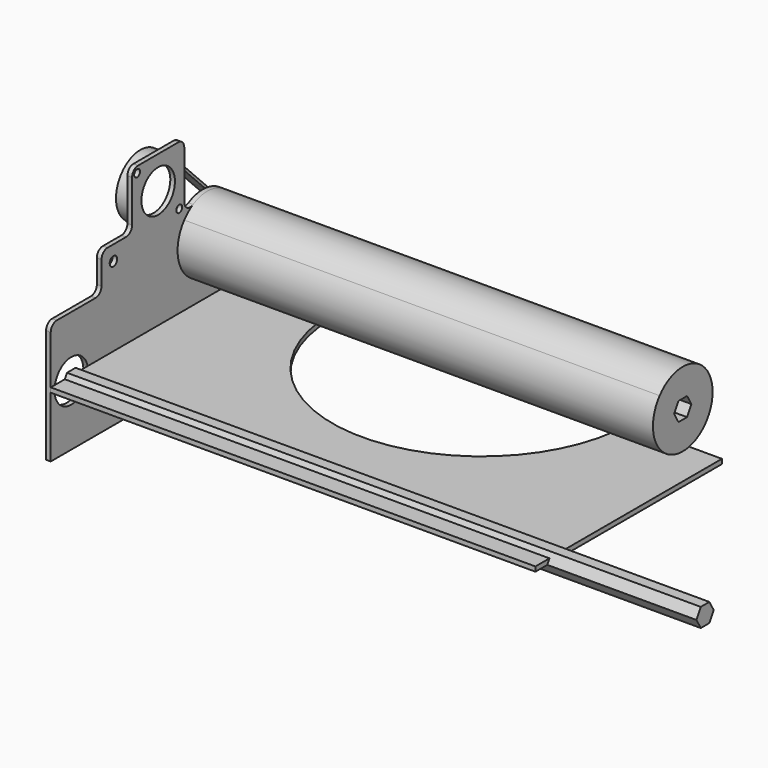
from build123d import *

# Parameters (mm, degrees)
F0_W     = 17.6947293282
F0_H     = 38.2016
F0_W_2   = 6.35
F0_H_2   = 28.575
F1_DEPTH = 3.175
F2_R     = 3.175
F2_R_2   = 2.4892
F2_R_3   = 14.2875
F3_DEPTH = 3.175
F4_R     = 14.2875
F5_DEPTH = 323.85
F6_DEPTH = 431.8
F8_DEPTH = 9
F9_R     = 5.08


# Not quite as in the source:
# - a feature names something its author has since deleted; it is built from what else it names


with BuildPart() as f1:
    # F0 (on Top) → F1 (new body)
    with BuildSketch(Plane.XY):
        with BuildLine():
            ThreePointArc((-90.5710140925, 31.75), (-98.622453308, 53.3708723969), (-101.5883780415, 76.2508))
            Line((-101.5883780415, 76.2508), (-147.4052706718, 76.2508))
            Line((-147.4052706718, 76.2508), (-147.4052706718, 38.0492))
            Line((-147.4052706718, 38.0492), (-165.1, 38.0492))
            Line((-165.1, 38.0492), (-165.1, 31.75))
            Line((-165.1, 31.75), (-90.5710140925, 31.75))
        make_face()
        with Locations((-156.2526353359, 57.15)):
            Rectangle(F0_W, F0_H)
        with BuildLine():
            Line((165.1, 76.2508), (101.5883780415, 76.2508))
            ThreePointArc((101.5883780415, 76.2508), (98.622453308, 53.3708723969), (90.5710140925, 31.75))
            Line((90.5710140925, 31.75), (165.1, 31.75))
            Line((165.1, 31.75), (165.1, 76.2508))
        make_face()
        with BuildLine():
            ThreePointArc((90.5710140925, 31.75), (0, -23.8125), (-90.5710140925, 31.75))
            Line((-90.5710140925, 31.75), (-165.1, 31.75))
            Line((-165.1, 31.75), (-165.1, -47.625))
            Line((-165.1, -47.625), (-158.75, -47.625))
            Line((-158.75, -47.625), (-158.75, -76.2))
            Line((-158.75, -76.2), (-165.1, -76.2))
            Line((-165.1, -76.2), (-165.1, -82.55))
            Line((-165.1, -82.55), (165.1, -82.55))
            Line((165.1, -82.55), (165.1, 31.75))
            Line((165.1, 31.75), (90.5710140925, 31.75))
        make_face()
        with Locations((-161.925, -61.9125)):
            Rectangle(F0_W_2, F0_H_2)
    extrude(amount=F1_DEPTH)


with BuildPart() as f3:
    # F2 (on face) → F3 (new body)
    with BuildSketch(Plane(origin=(-165.1, 0, 0), x_dir=(0, -1, 0), z_dir=(-1, 0, 0))):
        with BuildLine():
            Line((-31.1531, 41.275), (-36.5633, 41.275))
            ThreePointArc((-36.5633, 41.275), (-50.8508, 26.9875), (-65.1383, 41.275))
            Line((-65.1383, 41.275), (-76.2508, 41.275))
            ThreePointArc((-76.2508, 41.275), (-50.8508, 15.875), (-25.4508, 41.275))
            Line((-25.4508, 41.275), (-31.1531, 41.275))
        make_face()
        with BuildLine():
            Line((-31.1531, 57.3112281946), (-31.1531, 41.275))
            Line((-31.1531, 41.275), (-25.4508, 41.275))
            ThreePointArc((-25.4508, 41.275), (-26.9187965318, 49.7849477084), (-31.1531, 57.3112281946))
        make_face()
        with BuildLine():
            Line((50.8, 0), (-76.2508, 0))
            Line((-76.2508, 0), (-76.2508, -41.275))
            Line((-76.2508, -41.275), (76.2508, -41.275))
            Line((76.2508, -41.275), (76.2508, -8.9170280565))
            ThreePointArc((76.2508, -8.9170280565), (60.3632536315, -13.4838478373), (50.8, 0))
        make_face()
        with BuildLine():
            Line((76.2508, 41.275), (76.2508, 8.9170280565))
            ThreePointArc((76.2508, 8.9170280565), (77.9585667504, 6.2022815929), (79.017755965, 3.175))
            Line((79.017755965, 3.175), (82.55, 3.175))
            Line((82.55, 3.175), (82.55, 41.275))
            Line((82.55, 41.275), (76.2508, 41.275))
        make_face()
        with BuildLine():
            Line((76.2508, -8.9170280565), (76.2508, -41.275))
            Line((76.2508, -41.275), (82.55, -41.275))
            Line((82.55, -41.275), (82.55, 0))
            Line((82.55, 0), (79.375, 0))
            ThreePointArc((79.375, 0), (78.5713478373, -4.7242463685), (76.2508, -8.9170280565))
        make_face()
        Polygon((13.2969, 61.5398025967), (13.2969, 41.275), (39.3043012984, 41.275), (39.3043012984, 67.2824012984), (13.2969, 67.2824012984), align=None)
        with Locations((29.1719, 57.15)):
            Circle(F2_R, mode=Mode.SUBTRACT)
        with BuildLine():
            ThreePointArc((-31.1531, 57.3112281946), (-26.9187965318, 49.7849477084), (-25.4508, 41.275))
            Line((-25.4508, 41.275), (13.2969, 41.275))
            Line((13.2969, 41.275), (13.2969, 61.5398025967))
            Line((13.2969, 61.5398025967), (-31.1531, 61.5398025967))
            Line((-31.1531, 61.5398025967), (-31.1531, 57.3112281946))
        make_face()
        with BuildLine():
            Line((51.157244035, 3.175), (-76.2508, 3.175))
            Line((-76.2508, 3.175), (-76.2508, 0))
            Line((-76.2508, 0), (50.8, 0))
            ThreePointArc((50.8, 0), (50.8895919085, 1.5975174726), (51.157244035, 3.175))
        make_face()
        with BuildLine():
            Line((82.55, 3.175), (79.017755965, 3.175))
            ThreePointArc((79.017755965, 3.175), (79.2854080915, 1.5975174726), (79.375, 0))
            Line((79.375, 0), (82.55, 0))
            Line((82.55, 0), (82.55, 3.175))
        make_face()
        Polygon((-31.1531, 105.9898025967), (-31.1531, 61.5398025967), (13.2969, 61.5398025967), (13.2969, 67.2824012984), (13.2969, 73.025), (13.2969, 105.9898025967), align=None)
        with Locations((-26.8886122421, 65.8042903546)):
            Circle(F2_R_2, mode=Mode.SUBTRACT)
        with Locations((-8.9281, 83.7648025967)):
            Circle(F2_R_3, mode=Mode.SUBTRACT)
        with Locations((9.0324122421, 101.7253148389)):
            Circle(F2_R_2, mode=Mode.SUBTRACT)
        with BuildLine():
            Line((13.2969, 41.275), (-25.4508, 41.275))
            ThreePointArc((-25.4508, 41.275), (-50.8508, 15.875), (-76.2508, 41.275))
            Line((-76.2508, 41.275), (-76.2508, 3.175))
            Line((-76.2508, 3.175), (51.157244035, 3.175))
            ThreePointArc((51.157244035, 3.175), (61.9005370447, 13.9275239498), (76.2508, 8.9170280565))
            Line((76.2508, 8.9170280565), (76.2508, 41.275))
            Line((76.2508, 41.275), (45.0469, 41.275))
            Line((45.0469, 41.275), (39.3043012984, 41.275))
            Line((39.3043012984, 41.275), (13.2969, 41.275))
        make_face()
        with BuildLine():
            ThreePointArc((-65.1383, 41.275), (-50.8508, 55.5625), (-36.5633, 41.275))
            Line((-36.5633, 41.275), (-31.1531, 41.275))
            Line((-31.1531, 41.275), (-31.1531, 57.3112281946))
            ThreePointArc((-31.1531, 57.3112281946), (-59.3607477084, 65.2070034682), (-76.2508, 41.275))
            Line((-76.2508, 41.275), (-65.1383, 41.275))
        make_face()
    extrude(amount=F3_DEPTH)

    # F9
    f9_edges = [f3.edges().sort_by_distance(p)[0] for p in [
        (-166.6875, 76.2508, 41.275),
        (-166.6875, -39.304301, 41.275),
        (-166.6875, -82.55, 41.275),
        (-166.6875, -39.304301, 67.282401),
        (-166.6875, -13.2969, 67.282401),
        (-166.6875, -13.2969, 105.989803),
        (-166.6875, 31.1531, 105.989803),
        (-166.6875, 31.1531, 57.311228),
    ]]
    fillet(f9_edges, radius=F9_R)


with BuildPart() as f5:
    # F4 (on face) → F5 (new body)
    with BuildSketch(Plane.YZ.offset(-165.1)):
        with BuildLine():
            ThreePointArc((31.1531, 57.3112281946), (42.3408522916, 17.3429965318), (76.2508, 41.275))
            ThreePointArc((76.2508, 41.275), (59.3607477084, 65.2070034682), (31.1531, 57.3112281946))
        make_face()
        with Locations((50.8508, 41.275)):
            Circle(F4_R, mode=Mode.SUBTRACT)
        with Locations((50.8508, 41.275)):
            Circle(F4_R)
        Polygon((43.5184515813, 41.275), (47.1846257906, 47.625), (54.5169742094, 47.625), (58.1831484187, 41.275), (54.5169742094, 34.925), (47.1846257906, 34.925), align=None, mode=Mode.SUBTRACT)
    extrude(amount=F5_DEPTH)


with BuildPart() as f6:
    # F4 (on face) → F6 (new body)
    with BuildSketch(Plane.YZ.offset(-165.1)):
        Polygon((-61.4213257906, 6.35), (-68.7536742094, 6.35), (-72.4198484187, 0), (-68.7536742094, -6.35), (-61.4213257906, -6.35), (-57.7551515813, 0), align=None)
    extrude(amount=F6_DEPTH)


with BuildPart() as f8:
    # F7 (on face) → F8 (new body)
    with BuildSketch(Plane(origin=(-168.275, 0, 0), x_dir=(0, -1, 0), z_dir=(-1, 0, 0))):
        with BuildLine():
            ThreePointArc((-37.254063169, 27.859736), (-64.266064, 27.678263169), (-64.447536831, 54.690264))
            Line((-64.447536831, 54.690264), (-52.6884316676, 66.6084385715))
            ThreePointArc((-52.6884316676, 66.6084385715), (-53.9729276626, 66.4823861965), (-55.2493622465, 66.2912477235))
            Line((-55.2493622465, 66.2912477235), (-65.5866251559, 55.8141491489))
            ThreePointArc((-65.5866251559, 55.8141491489), (-65.3899491489, 26.5391748441), (-36.1149748441, 26.7358508511))
            Line((-36.1149748441, 26.7358508511), (5.8077251559, 69.2256534478))
            ThreePointArc((5.8077251559, 69.2256534478), (5.6110491489, 98.5006277526), (-23.6639251559, 98.3039517457))
            Line((-23.6639251559, 98.3039517457), (-31.1531, 90.7134682907))
            Line((-31.1531, 90.7134682907), (-31.1531, 88.4350859823))
            Line((-31.1531, 88.4350859823), (-22.524836831, 97.1800665967))
            ThreePointArc((-22.524836831, 97.1800665967), (4.487164, 97.3615394277), (4.668636831, 70.3495385967))
            Line((4.668636831, 70.3495385967), (-37.254063169, 27.859736))
        make_face()
        with BuildLine():
            ThreePointArc((-55.2493622465, 66.2912477235), (-53.9729276626, 66.4823861965), (-52.6884316676, 66.6084385715))
            Line((-52.6884316676, 66.6084385715), (-31.1531, 88.4350859823))
            Line((-31.1531, 88.4350859823), (-31.1531, 90.7134682907))
            Line((-31.1531, 90.7134682907), (-55.2493622465, 66.2912477235))
        make_face()
    extrude(amount=F8_DEPTH)


solid = Compound([f1.part, f3.part, f5.part, f6.part, f8.part])
